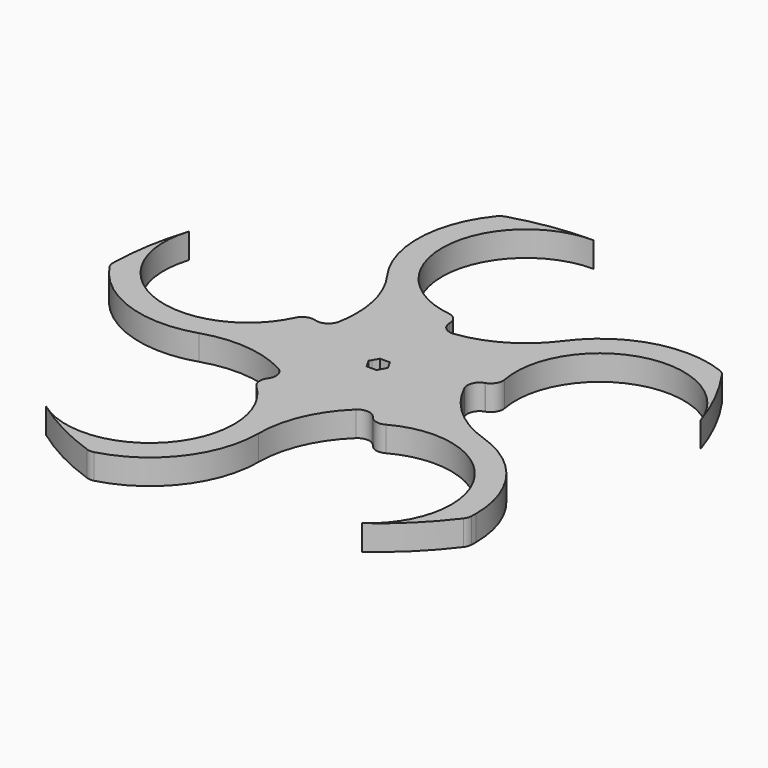
from build123d import *

# Parameters (mm, degrees)
F1_DEPTH    = 19.05
F2_T1_DEPTH = 19.05
F2_T3_DEPTH = 33.4673134048
F2_T5_DEPTH = 62.4401148549


# Not quite as in the source:
# - a fillet or chamfer that OpenCascade refuses, or shapes differently, is made with other operations: its cross-section is extruded or revolved along the edge and cut away or added


with BuildPart() as f1:
    # F0 (on Top) → F1 (new body)
    with BuildSketch(Plane.XY):
        with BuildLine():
            ThreePointArc((119.4379632658, -164.392253257), (143.4023261419, -143.965318244), (163.9230028488, -120.0811772803))
            ThreePointArc((163.9230028488, -120.0811772803), (164.1511150811, -116.5537002375), (164.2271994905, -113.0196741142))
            ThreePointArc((164.2271994905, -113.0196741142), (148.5448974992, -64.7545112961), (107.4880978294, -34.9250000954))
            ThreePointArc((107.4880978294, -34.9250000954), (69.268202849, -31.9170290174), (33.8484368023, -46.588376451))
            Line((33.8484368023, -46.588376451), (44.7892362247, -61.6470949714))
            ThreePointArc((44.7892362247, -61.6470949714), (110.9419964787, -56.4407598282), (145.6135997453, -113.0196741142))
            ThreePointArc((145.6135997453, -113.0196741142), (138.6925140312, -141.8480708476), (119.4379632658, -164.392253257))
        make_face()
        with BuildLine():
            ThreePointArc((72.4705065417, 23.5470949714), (113.2400161836, 103.5617628989), (193.2546841112, 62.792253257))
            ThreePointArc((193.2546841112, 62.792253257), (181.2329098472, 91.8959867911), (164.8589797861, 118.7929155459))
            ThreePointArc((164.8589797861, 118.7929155459), (110.8726675576, 122.284061806), (66.4312977521, 91.4348371795))
            ThreePointArc((66.4312977521, 91.4348371795), (51.7599502656, 56.0150712376), (54.7679212123, 17.7951763236))
            Line((54.7679212123, 17.7951763236), (72.4705065417, 23.5470949714))
        make_face()
        with BuildLine():
            ThreePointArc((33.8484368023, -46.588376451), (69.268202849, -31.9170290174), (107.4880978294, -34.9250000954))
            ThreePointArc((107.4880978294, -34.9250000954), (74.799512228, -14.8934092025), (54.7679212123, 17.7951763236))
            Line((54.7679212123, 17.7951763236), (6.1741283973, 2.0060959234))
            Line((6.1741283973, 2.0060959234), (7.3323484187, 0))
            Line((7.3323484187, 0), (4.0856602382, -5.623428885))
            Line((4.0856602382, -5.623428885), (33.8484368023, -46.588376451))
        make_face()
        with BuildLine():
            ThreePointArc((0, -113.0196741142), (8.9498466476, -75.7408799304), (33.8484368023, -46.588376451))
            Line((33.8484368023, -46.588376451), (4.0856602382, -5.623428885))
            Line((4.0856602382, -5.623428885), (3.6661742094, -6.35))
            Line((3.6661742094, -6.35), (-3.6661742094, -6.35))
            Line((-3.6661742094, -6.35), (-4.0856602382, -5.623428885))
            Line((-4.0856602382, -5.623428885), (-33.8484368023, -46.588376451))
            ThreePointArc((-33.8484368023, -46.588376451), (-8.9498466476, -75.7408799304), (0, -113.0196741142))
        make_face()
        with BuildLine():
            Line((6.1741283973, 2.0060959234), (54.7679212123, 17.7951763236))
            ThreePointArc((54.7679212123, 17.7951763236), (51.7599502656, 56.0150712376), (66.4312977521, 91.4348371795))
            ThreePointArc((66.4312977521, 91.4348371795), (37.2787942512, 66.5362469367), (0, 57.5864002547))
            Line((0, 57.5864002547), (0, 6.35))
            Line((0, 6.35), (3.6661742094, 6.35))
            Line((3.6661742094, 6.35), (6.1741283973, 2.0060959234))
        make_face()
        with BuildLine():
            ThreePointArc((-119.4379632658, -164.392253257), (-92.6053982257, -180.8714466671), (-63.5489924876, -193.0071645142))
            ThreePointArc((-63.5489924876, -193.0071645142), (-17.8211040988, -164.0992029557), (0, -113.0196741142))
            ThreePointArc((0, -113.0196741142), (-8.9498466476, -75.7408799304), (-33.8484368023, -46.588376451))
            Line((-33.8484368023, -46.588376451), (-44.7892362247, -61.6470949714))
            ThreePointArc((-44.7892362247, -61.6470949714), (-25.5346854593, -84.1912773807), (-18.6135997453, -113.0196741142))
            ThreePointArc((-18.6135997453, -113.0196741142), (-53.2852030118, -169.5985884001), (-119.4379632658, -164.392253257))
        make_face()
        with BuildLine():
            ThreePointArc((-107.4880971788, -34.924999884), (-69.2682025112, -31.9170290709), (-33.8484368023, -46.588376451))
            Line((-33.8484368023, -46.588376451), (-4.0856602382, -5.623428885))
            Line((-4.0856602382, -5.623428885), (-7.3323484187, 0))
            Line((-7.3323484187, 0), (-6.1741283973, 2.0060959234))
            Line((-6.1741283973, 2.0060959234), (-54.7679212123, 17.7951763236))
            ThreePointArc((-54.7679212123, 17.7951763236), (-74.7995119862, -14.8934089606), (-107.4880971788, -34.924999884))
        make_face()
        with BuildLine():
            ThreePointArc((0, 76.2), (-63.5, 139.7), (0, 203.2))
            ThreePointArc((0, 203.2), (-31.3942279763, 200.7601615106), (-62.0345499904, 193.4992367104))
            ThreePointArc((-62.0345499904, 193.4992367104), (-82.037515312, 143.2340266773), (-66.431298315, 91.4348379542))
            ThreePointArc((-66.431298315, 91.4348379542), (-37.2787946778, 66.5362471541), (0, 57.5864002547))
            Line((0, 57.5864002547), (0, 76.2))
        make_face()
        with BuildLine():
            Line((0, 6.35), (0, 57.5864002547))
            ThreePointArc((0, 57.5864002547), (-37.2787946778, 66.5362471541), (-66.431298315, 91.4348379542))
            ThreePointArc((-66.431298315, 91.4348379542), (-54.7679213836, 68.5441724321), (-50.7489955812, 43.1696741142))
            ThreePointArc((-50.7489955812, 43.1696741142), (-51.7599502537, 30.3242770655), (-54.7679212123, 17.7951763236))
            Line((-54.7679212123, 17.7951763236), (-6.1741283973, 2.0060959234))
            Line((-6.1741283973, 2.0060959234), (-3.6661742094, 6.35))
            Line((-3.6661742094, 6.35), (0, 6.35))
        make_face()
        with BuildLine():
            ThreePointArc((-193.2546841112, 62.792253257), (-200.6356097871, 32.1806166093), (-203.198440157, 0.7961895383))
            ThreePointArc((-203.198440157, 0.7961895383), (-161.574640139, -33.7605653616), (-107.4880971788, -34.924999884))
            ThreePointArc((-107.4880971788, -34.924999884), (-74.7995119862, -14.8934089606), (-54.7679212123, 17.7951763236))
            Line((-54.7679212123, 17.7951763236), (-72.4705065417, 23.5470949714))
            ThreePointArc((-72.4705065417, 23.5470949714), (-152.4851744692, -17.2224146706), (-193.2546841112, 62.792253257))
        make_face()
    extrude(amount=F1_DEPTH)

    # F2: fillet of radius 9.271 on 18 edges, made by hand

    # F2_s2 → F2_t1 (join)
    with BuildSketch(Plane.XY):
        with BuildLine():
            ThreePointArc((-52.1734982583, 27.9409881084), (-56.556536878, 21.6850582504), (-64.1485619626, 20.8431312667))
            Line((-64.1485619626, 20.8431312667), (-54.7679212123, 17.7951763236))
            ThreePointArc((-54.7679212123, 17.7951763236), (-53.3088030101, 22.8266804501), (-52.1734982583, 27.9409881084))
        make_face()
        with BuildLine():
            ThreePointArc((10.4509611944, 58.2541856616), (3.146784917, 60.4895144603), (0, 67.4497896429))
            Line((0, 67.4497896429), (0, 57.5864002547))
            ThreePointArc((0, 57.5864002547), (5.2361371076, 57.7535166629), (10.4509611944, 58.2541856616))
        make_face()
        with BuildLine():
            ThreePointArc((58.6325474916, 8.0620786174), (58.501356912, 15.6995176491), (64.1485619626, 20.8431312667))
            Line((64.1485619626, 20.8431312667), (54.7679212123, 17.7951763236))
            ThreePointArc((54.7679212123, 17.7951763236), (56.5449137123, 12.8669558174), (58.6325474916, 8.0620786174))
        make_face()
        with BuildLine():
            ThreePointArc((25.7859460024, -53.2715470561), (33.0090420427, -50.7866789462), (39.6459916223, -54.5680260881))
            Line((39.6459916223, -54.5680260881), (33.8484368023, -46.588376451))
            ThreePointArc((33.8484368023, -46.588376451), (29.7105414576, -49.801300636), (25.7859460024, -53.2715470561))
        make_face()
        with BuildLine():
            ThreePointArc((-42.6959564301, -40.9857053314), (-38.1006469936, -47.0874114136), (-39.6459916223, -54.5680260881))
            Line((-39.6459916223, -54.5680260881), (-33.8484368023, -46.588376451))
            ThreePointArc((-33.8484368023, -46.588376451), (-38.1827892674, -43.6458522944), (-42.6959564301, -40.9857053314))
        make_face()
    extrude(amount=F2_T1_DEPTH)

    # F2_s4 → F2_t3 (cut)
    with BuildSketch(Plane.XY.offset(-7.2086567024)):
        with BuildLine():
            ThreePointArc((-66.1835050247, -192.1197118014), (-63.4817465047, -192.6197992349), (-60.7520682549, -192.3060426495))
            ThreePointArc((-60.7520682549, -192.3060426495), (-62.1474526007, -192.6688814632), (-63.5489924876, -193.0071645142))
            ThreePointArc((-63.5489924876, -193.0071645142), (-64.8677664235, -192.56794354), (-66.1835050247, -192.1197118014))
        make_face()
        with BuildLine():
            ThreePointArc((162.2648760175, -122.3125096261), (163.5753767273, -119.8975200957), (164.1204934505, -117.2044856919))
            ThreePointArc((164.1204934505, -117.2044856919), (164.0343761921, -118.6436984264), (163.9230028488, -120.0811772803))
            ThreePointArc((163.9230028488, -120.0811772803), (163.0977553213, -121.1996790803), (162.2648760175, -122.3125096261))
        make_face()
        with BuildLine():
            ThreePointArc((166.4687135838, 116.5264236032), (164.5768890447, 118.5190566489), (162.1841114577, 119.8696868579))
            ThreePointArc((162.1841114577, 119.8696868579), (163.5262724108, 119.3430432847), (164.8589797861, 118.7929155459))
            ThreePointArc((164.8589797861, 118.7929155459), (165.6677227009, 117.6624224428), (166.4687135838, 116.5264236032))
        make_face()
        with BuildLine():
            ThreePointArc((-59.3815529592, 194.3298000003), (-61.8612655349, 193.1463254193), (-63.8852001344, 191.2880263909))
            ThreePointArc((-63.8852001344, 191.2880263909), (-62.9695817887, 192.4017554972), (-62.0345499904, 193.4992367104))
            ThreePointArc((-62.0345499904, 193.4992367104), (-60.7094718533, 193.9190553486), (-59.3815529592, 194.3298000003))
        make_face()
        with BuildLine():
            ThreePointArc((-203.1685316174, 3.575997824), (-202.8092537324, 0.8519372624), (-201.6673365189, -1.6471849074))
            ThreePointArc((-201.6673365189, -1.6471849074), (-202.4436142136, -0.4322188923), (-203.198440157, 0.7961895383))
            ThreePointArc((-203.198440157, 0.7961895383), (-203.1882397453, 2.1861448289), (-203.1685316174, 3.575997824))
        make_face()
    extrude(amount=F2_T3_DEPTH, mode=Mode.SUBTRACT)

    # F2_s6 → F2_t5 (cut)
    with BuildSketch(Plane.XY.offset(-21.6950574275)):
        with BuildLine():
            ThreePointArc((51.638223753, -57.3105953376), (45.1569902325, -58.2226827749), (39.6884223033, -54.6264269103))
            Line((39.6884223033, -54.6264269103), (44.7892362247, -61.6470949714))
            ThreePointArc((44.7892362247, -61.6470949714), (48.14445968, -59.3694409066), (51.638223753, -57.3105953376))
        make_face()
        with BuildLine():
            ThreePointArc((64.2172162466, 20.8654383958), (69.3273392459, 24.9550513813), (70.4627038476, 31.4009212731))
            ThreePointArc((70.4627038476, 31.4009212731), (71.3411498691, 27.4419359155), (72.4705065417, 23.5470949714))
            Line((72.4705065417, 23.5470949714), (64.2172162466, 20.8654383958))
        make_face()
        with BuildLine():
            ThreePointArc((0, 67.521977029), (-2.3103382289, 73.6457527196), (-8.089877836, 76.7174319625))
            ThreePointArc((-8.089877836, 76.7174319625), (-4.0532042644, 76.3294900195), (0, 76.2))
            Line((0, 76.2), (0, 67.521977029))
        make_face()
        with BuildLine():
            ThreePointArc((-64.2172162466, 20.8654383958), (-70.7552067969, 20.5605269264), (-75.4625233151, 16.0130592093))
            ThreePointArc((-75.4625233151, 16.0130592093), (-73.8461678679, 19.7322832604), (-72.4705065417, 23.5470949714))
            Line((-72.4705065417, 23.5470949714), (-64.2172162466, 20.8654383958))
        make_face()
        with BuildLine():
            ThreePointArc((-39.6884223033, -54.6264269103), (-41.4187844526, -60.9386482525), (-38.5485264496, -66.8208171073))
            ThreePointArc((-38.5485264496, -66.8208171073), (-41.5862374169, -64.1342682889), (-44.7892362247, -61.6470949714))
            Line((-44.7892362247, -61.6470949714), (-39.6884223033, -54.6264269103))
        make_face()
    extrude(amount=F2_T5_DEPTH, mode=Mode.SUBTRACT)


solid = f1.part
